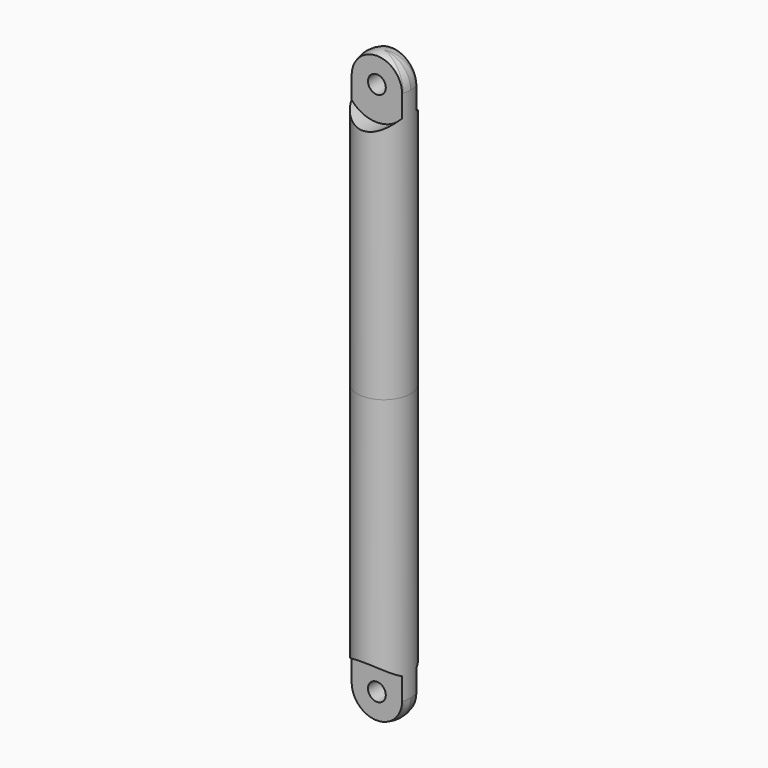
from build123d import *

# Parameters (mm, degrees)
F0_R        = 6
F1_DEPTH    = 66
F3_START    = -2
F3_DEPTH    = 4.0010001005
F4_START    = 2
F4_DEPTH    = 4
F5_T2_ANGLE = 325.4381048425
F5_T4_ANGLE = 162.7109745837
F5_T6_ANGLE = 162.7109745837
F6_R        = 2
F7_DEPTH    = 12.5
F8_R        = 4.8
F9_DEPTH    = 6
F10_R       = 2.375
F11_DEPTH   = 7.5


# Not quite as in the source:
# - a fillet or chamfer that OpenCascade refuses, or shapes differently, is made with other operations: its cross-section is extruded or revolved along the edge and cut away or added


with BuildPart() as f1:
    # F0 (on Top) → F1 (new body)
    with BuildSketch(Plane.XY):
        Circle(F0_R)
    extrude(amount=F1_DEPTH)

    # F2 (on Front) → F3 (cut)
    with BuildSketch(Plane.XZ.offset(F3_START)):
        with BuildLine():
            Line((-6.0225790367, 66.0244730711), (-6.0225790367, 55.5302637944))
            ThreePointArc((-6.0225790367, 55.5302637944), (0.1221735447, 52.5009951577), (6.1649857089, 55.7288232056))
            Line((6.1649857089, 55.7288232056), (6.1649857089, 66.0244730711))
            Line((6.1649857089, 66.0244730711), (-6.0225790367, 66.0244730711))
        make_face()
    extrude(amount=-F3_DEPTH, mode=Mode.SUBTRACT)

    # F2 (on Front) → F4 (cut)
    with BuildSketch(Plane.XZ.offset(F4_START)):
        with BuildLine():
            Line((-6.0225790367, 66.0244730711), (-6.0225790367, 55.5302637944))
            ThreePointArc((-6.0225790367, 55.5302637944), (0.1221735447, 52.5009951577), (6.1649857089, 55.7288232056))
            Line((6.1649857089, 55.7288232056), (6.1649857089, 66.0244730711))
            Line((6.1649857089, 66.0244730711), (-6.0225790367, 66.0244730711))
        make_face()
    extrude(amount=F4_DEPTH, mode=Mode.SUBTRACT)

    # F5: fillet of radius 6 on 3 edges, made by hand

    # F5_s1 → F5_t2 (revolve, cut)
    with BuildSketch(Plane(origin=(0, 0, 0), x_dir=(0, 0, 1), z_dir=(0.2970573734, -0.954859632, 0))):
        with BuildLine():
            ThreePointArc((60.0001, -6.0001), (64.2427406871, -4.2427406871), (66.0001, -0.0001))
            Line((66.0001, -0.0001), (66.1201, -0.0001))
            ThreePointArc((66.1201, -0.0001), (66.12, -3.00005), (66.12, -6))
            Line((66.12, -6), (66, -6.12))
            ThreePointArc((66, -6.12), (63.00005, -6.12), (60.0001, -6.1201))
            Line((60.0001, -6.1201), (60.0001, -6.0001))
        make_face()
    revolve(axis=Axis((0, 0, 66), (0, 0, 1)), revolution_arc=F5_T2_ANGLE, mode=Mode.SUBTRACT)

    # F5_s3 → F5_t4 (revolve, cut)
    with BuildSketch(Plane.XZ):
        with BuildLine():
            ThreePointArc((6.0001, 60.0001), (4.2427406871, 64.2427406871), (0.0001, 66.0001))
            Line((0.0001, 66.0001), (0.0001, 66.1201))
            ThreePointArc((0.0001, 66.1201), (3.00005, 66.12), (6, 66.12))
            Line((6, 66.12), (6.12, 66))
            ThreePointArc((6.12, 66), (6.12, 63.00005), (6.1201, 60.0001))
            Line((6.1201, 60.0001), (6.0001, 60.0001))
        make_face()
    revolve(axis=Axis((0, 0, 66), (0, 0, 1)), revolution_arc=F5_T4_ANGLE, mode=Mode.SUBTRACT)

    # F5_s5 → F5_t6 (revolve, cut)
    with BuildSketch(Plane(origin=(0, 0, 0), x_dir=(0, 0, 1), z_dir=(-0.2971919912, 0.954817742, 0))):
        with BuildLine():
            ThreePointArc((60.0001, -6.0001), (64.2427406871, -4.2427406871), (66.0001, -0.0001))
            Line((66.0001, -0.0001), (66.1201, -0.0001))
            ThreePointArc((66.1201, -0.0001), (66.12, -3.00005), (66.12, -6))
            Line((66.12, -6), (66, -6.12))
            ThreePointArc((66, -6.12), (63.00005, -6.12), (60.0001, -6.1201))
            Line((60.0001, -6.1201), (60.0001, -6.0001))
        make_face()
    revolve(axis=Axis((0, 0, 66), (0, 0, 1)), revolution_arc=F5_T6_ANGLE, mode=Mode.SUBTRACT)

    # F6 (on face) → F7 (cut, symmetric)
    with BuildSketch(Plane.XZ):
        with Locations((0, 60)):
            Circle(F6_R)
    extrude(amount=F7_DEPTH, both=True, mode=Mode.SUBTRACT)

    # F8 (on face) → F9 (cut)
    with BuildSketch(Plane(origin=(0, 0, 0), x_dir=(1, 0, 0), z_dir=(0, 0, -1))):
        Circle(F8_R)
    extrude(amount=-F9_DEPTH, mode=Mode.SUBTRACT)

    # F10 (on face) → F11 (join)
    with BuildSketch(Plane(origin=(0, 0, 6), x_dir=(1, 0, 0), z_dir=(0, 0, -1))):
        Circle(F10_R)
    extrude(amount=F11_DEPTH)

    # F12: F1 across plane


with BuildPart() as f1_1:
    add(f1.part)
    add(f1.part.mirror(Plane.XY))


solid = f1_1.part
